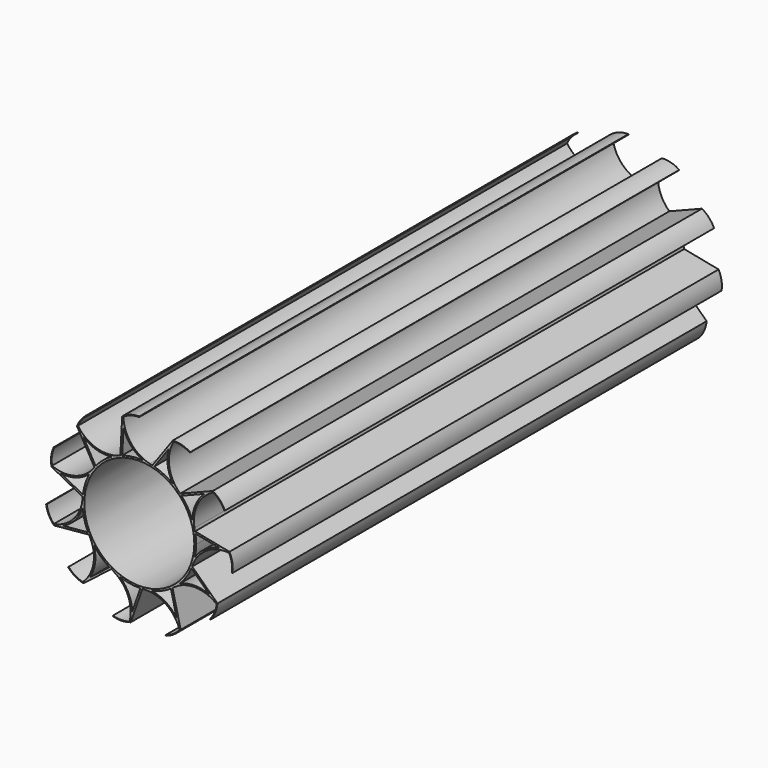
from build123d import *

# Parameters (mm, degrees)
F0_R          = 450
F1_DEPTH      = 5000
F4_DEPTH      = 7
F4_DEPTH_BACK = 7


# Not quite as in the source:
# - a feature names something its author has since deleted; it is built from what else it names


with BuildPart() as f1:
    # F0 (on Front) → F1 (new body)
    with BuildSketch(Plane.XZ):
        with BuildLine():
            ThreePointArc((29.6722661009, 464.0523209989), (57.272095407, 461.4595400332), (84.6683771855, 457.226711714))
            ThreePointArc((84.6683771855, 457.226711714), (-67.5951607035, 555.0944140008), (-130, 725))
            ThreePointArc((-130, 725), (-68.0073525437, 754.773895767), (0, 765))
            Line((0, 765), (0, 770))
            ThreePointArc((0, 770), (-73.5272058493, 758.4735293088), (-140, 725))
            Line((-140, 725), (-154.7293809103, 438.5017886886))
            ThreePointArc((-154.7293809103, 438.5017886886), (-147.110538763, 441.1161858115), (-139.4475537059, 443.5982188484))
            Line((-139.4475537059, 443.5982188484), (-129.0431979691, 645.9712395866))
            ThreePointArc((-129.0431979691, 645.9712395866), (-68.9398579749, 538.2132538291), (29.6722661009, 464.0523209989))
        make_face()
        with BuildLine():
            ThreePointArc((455.106133728, -95.4117762291), (462.5199196702, -47.9616920912), (465, 0))
            ThreePointArc((465, 0), (463.4796356702, 37.5716291765), (458.9284846496, 74.8975699022))
            ThreePointArc((458.9284846496, 74.8975699022), (457.5622716093, 82.8357869508), (456.0587595675, 90.7491477743))
            ThreePointArc((456.0587595675, 90.7491477743), (453.3481669029, 101.785731934), (451.0805611151, 112.9217755089))
            ThreePointArc((451.0805611151, 112.9217755089), (443.550050434, 139.6006903996), (434.4431435072, 165.7834583413))
            ThreePointArc((434.4431435072, 165.7834583413), (396.7252572047, 242.5573546522), (345.5825256109, 311.1233163753))
            ThreePointArc((345.5825256109, 311.1233163753), (340.1414699099, 317.0627389769), (334.5983492287, 322.9070217469))
            ThreePointArc((334.5983492287, 322.9070217469), (326.3512256914, 330.7261301277), (318.4229946099, 338.86840588))
            ThreePointArc((318.4229946099, 338.86840588), (297.66421554, 357.2408358334), (275.8475248515, 374.3436162583))
            ThreePointArc((275.8475248515, 374.3436162583), (202.6101176878, 418.5380988758), (122.5165564603, 448.5696081915))
            ThreePointArc((122.5165564603, 448.5696081915), (114.7281548389, 450.6245116361), (106.9053271687, 452.5441978668))
            ThreePointArc((106.9053271687, 452.5441978668), (95.7400762106, 454.6633188049), (84.6683771855, 457.226711714))
            ThreePointArc((84.6683771855, 457.226711714), (57.272095407, 461.4595400332), (29.6722661009, 464.0523209989))
            ThreePointArc((29.6722661009, 464.0523209989), (-55.8323026203, 461.6359539552), (-139.4475537059, 443.5982188484))
            ThreePointArc((-139.4475537059, 443.5982188484), (-147.110538763, 441.1161858115), (-154.7293809103, 438.5017886886))
            ThreePointArc((-154.7293809103, 438.5017886886), (-165.2678710001, 434.2481162591), (-175.9678517572, 430.4187671883))
            ThreePointArc((-175.9678517572, 430.4187671883), (-201.3035103525, 419.1681007899), (-225.9237274825, 406.4276926593))
            ThreePointArc((-225.9237274825, 406.4276926593), (-296.5483613387, 358.1676554176), (-357.1380508598, 297.7875293361))
            ThreePointArc((-357.1380508598, 297.7875293361), (-362.2426757411, 291.5565877697), (-367.238603816, 285.2381599073))
            ThreePointArc((-367.238603816, 285.2381599073), (-373.8044368952, 275.9622050517), (-380.7355310964, 266.9559052741))
            ThreePointArc((-380.7355310964, 266.9559052741), (-395.9666739177, 243.793751246), (-409.790533891, 219.7651435813))
            ThreePointArc((-409.790533891, 219.7651435813), (-443.1124106426, 140.9836569767), (-461.4397402826, 57.4314033257))
            ThreePointArc((-461.4397402826, 57.4314033257), (-462.3653226558, 49.4298331515), (-463.152164794, 41.413430752))
            ThreePointArc((-463.152164794, 41.413430752), (-463.6607352521, 30.060243596), (-464.6223694612, 18.7364296556))
            ThreePointArc((-464.6223694612, 18.7364296556), (-464.9132162808, -8.9833917542), (-463.5517412306, -36.6712857975))
            ThreePointArc((-463.5517412306, -36.6712857975), (-448.9914004502, -120.9616564115), (-419.237572543, -201.1587874497))
            ThreePointArc((-419.237572543, -201.1587874497), (-415.6902465446, -208.3905442378), (-412.0181859267, -215.5597700538))
            ThreePointArc((-412.0181859267, -215.5597700538), (-406.3080262366, -225.3856328058), (-400.9948883869, -235.4317299933))
            ThreePointArc((-400.9948883869, -235.4317299933), (-386.2530973946, -258.908371346), (-370.1385460296, -281.4648410425))
            ThreePointArc((-370.1385460296, -281.4648410425), (-312.3187930364, -344.5024985632), (-243.9304377122, -395.8824845298))
            ThreePointArc((-243.9304377122, -395.8824845298), (-237.0364542824, -400.0483962488), (-230.0713442091, -404.09426694))
            ThreePointArc((-230.0713442091, -404.09426694), (-219.9553897263, -409.2731632906), (-210.0543635442, -414.8519788504))
            ThreePointArc((-210.0543635442, -414.8519788504), (-184.9603492196, -426.6317723946), (-159.2089777382, -436.895297992))
            ThreePointArc((-159.2089777382, -436.895297992), (-76.4871755728, -458.6662315594), (8.8228875621, -464.9162899438))
            ThreePointArc((8.8228875621, -464.9162899438), (16.874737395, -464.6937090578), (24.9215236884, -464.3316892665))
            ThreePointArc((24.9215236884, -464.3316892665), (36.2315288916, -463.2193562166), (47.5769375506, -462.5596556265))
            ThreePointArc((47.5769375506, -462.5596556265), (75.0560029652, -458.902600144), (102.2683160682, -453.6145847838))
            ThreePointArc((102.2683160682, -453.6145847838), (183.6285797026, -427.2066768163), (258.775008375, -386.3424582421))
            ThreePointArc((258.775008375, -386.3424582421), (265.4283191806, -381.8020526097), (272.001983902, -377.1470810617))
            ThreePointArc((272.001983902, -377.1470810617), (280.9151930861, -370.0966764954), (290.1028971356, -363.4079100316))
            ThreePointArc((290.1028971356, -363.4079100316), (311.242604529, -345.4750947984), (331.2761421164, -326.3144459942))
            ThreePointArc((331.2761421164, -326.3144459942), (385.4435583801, -260.1120206821), (426.5678924457, -185.1076258139))
            ThreePointArc((426.5678924457, -185.1076258139), (429.7102850532, -177.6909421425), (432.7237361008, -170.2209394138))
            ThreePointArc((432.7237361008, -170.2209394138), (436.4102683277, -159.4709169651), (440.5232366492, -148.8767207192))
            ThreePointArc((440.5232366492, -148.8767207192), (448.61187829, -122.3616878648), (455.106133728, -95.4117762291))
        make_face()
        Circle(F0_R, mode=Mode.SUBTRACT)
        with BuildLine():
            ThreePointArc((456.0587595675, 90.7491477743), (457.5622716093, 82.8357869508), (458.9284846496, 74.8975699022))
            Line((458.9284846496, 74.8975699022), (657.7609456305, 35.7984317878))
            ThreePointArc((657.7609456305, 35.7984317878), (542.5461836828, -8.3575825515), (455.106133728, -95.4117762291))
            ThreePointArc((455.106133728, -95.4117762291), (448.61187829, -122.3616878648), (440.5232366492, -148.8767207192))
            ThreePointArc((440.5232366492, -148.8767207192), (559.0641476099, -12.0910323233), (736.1214743392, 25.4985296964))
            ThreePointArc((736.1214743392, 25.4985296964), (756.7698411808, -40.1003891557), (757.2134030389, -108.8708512791))
            Line((757.2134030389, -108.8708512791), (762.1625102483, -109.5824254704))
            ThreePointArc((762.1625102483, -109.5824254704), (761.2173748181, -35.163232747), (737.5446227219, 35.3967441152))
            Line((737.5446227219, 35.3967441152), (456.0587595675, 90.7491477743))
        make_face()
        with BuildLine():
            ThreePointArc((434.4431435072, 165.7834583413), (443.550050434, 139.6006903996), (451.0805611151, 112.9217755089))
            ThreePointArc((451.0805611151, 112.9217755089), (476.8515948552, 292.0812741164), (605.4792449418, 419.4280438225))
            ThreePointArc((605.4792449418, 419.4280438225), (658.3152096068, 375.4060715166), (695.8684764462, 317.7924849464))
            Line((695.8684764462, 317.7924849464), (700.416636423, 319.8695600115))
            ThreePointArc((700.416636423, 319.8695600115), (659.3874847149, 381.9639900089), (601.3250948118, 428.524363776))
            Line((601.3250948118, 428.524363776), (334.5983492287, 322.9070217469))
            ThreePointArc((334.5983492287, 322.9070217469), (340.1414699099, 317.0627389769), (345.5825256109, 311.1233163753))
            Line((345.5825256109, 311.1233163753), (533.9896258446, 385.7279725473))
            ThreePointArc((533.9896258446, 385.7279725473), (460.9373440098, 286.2917664064), (434.4431435072, 165.7834583413))
        make_face()
        with BuildLine():
            Line((639.5989441592, -368.9690917007), (432.7237361008, -170.2209394138))
            ThreePointArc((432.7237361008, -170.2209394138), (429.7102850532, -177.6909421425), (426.5678924457, -185.1076258139))
            Line((426.5678924457, -185.1076258139), (572.6978126954, -325.4968581247))
            ThreePointArc((572.6978126954, -325.4968581247), (451.9004434847, -300.353458101), (331.2761421164, -326.3144459942))
            ThreePointArc((331.2761421164, -326.3144459942), (311.242604529, -345.4750947984), (290.1028971356, -363.4079100316))
            ThreePointArc((290.1028971356, -363.4079100316), (463.777783657, -312.4245214315), (633.0503368197, -376.5265874443))
            ThreePointArc((633.0503368197, -376.5265874443), (614.95539526, -442.8752596068), (578.148424381, -500.9684614681))
            Line((578.148424381, -500.9684614681), (581.9271722528, -504.2427651379))
            ThreePointArc((581.9271722528, -504.2427651379), (621.3661269215, -441.1263775572), (639.5989441592, -368.9690917007))
        make_face()
        with BuildLine():
            Line((338.5851200161, -656.1898479127), (272.001983902, -377.1470810617))
            ThreePointArc((272.001983902, -377.1470810617), (265.4283191806, -381.8020526097), (258.775008375, -386.3424582421))
            Line((258.775008375, -386.3424582421), (305.8071707189, -583.4491954336))
            ThreePointArc((305.8071707189, -583.4491954336), (217.7795054561, -496.9892328997), (102.2683160682, -453.6145847838))
            ThreePointArc((102.2683160682, -453.6145847838), (75.0560029652, -458.902600144), (47.5769375506, -462.5596556265))
            ThreePointArc((47.5769375506, -462.5596556265), (221.2452502902, -513.5654324714), (328.9901902799, -659.0071734811))
            ThreePointArc((328.9901902799, -659.0071734811), (277.8969564114, -705.0403643399), (215.5254059837, -734.0121248151))
            Line((215.5254059837, -734.0121248151), (216.9340687679, -738.8095896832))
            ThreePointArc((216.9340687679, -738.8095896832), (284.2355240906, -707.0350143431), (338.5851200161, -656.1898479127))
        make_face()
        with BuildLine():
            Line((-69.927087404, -735.0749638283), (24.9215236884, -464.3316892665))
            ThreePointArc((24.9215236884, -464.3316892665), (16.874737395, -464.6937090578), (8.8228875621, -464.9162899438))
            Line((8.8228875621, -464.9162899438), (-58.1750872306, -656.1605356472))
            ThreePointArc((-58.1750872306, -656.1605356472), (-85.4848867983, -535.8344378108), (-159.2089777382, -436.895297992))
            ThreePointArc((-159.2089777382, -436.895297992), (-184.9603492196, -426.6317723946), (-210.0543635442, -414.8519788504))
            ThreePointArc((-210.0543635442, -414.8519788504), (-91.5310867995, -551.6529473815), (-79.5220171402, -732.2576382599))
            ThreePointArc((-79.5220171402, -732.2576382599), (-147.3918025718, -743.3601349722), (-215.5254059837, -734.0121248151))
            Line((-215.5254059837, -734.0121248151), (-216.9340687679, -738.8095896832))
            ThreePointArc((-216.9340687679, -738.8095896832), (-143.1378493268, -748.4650297457), (-69.927087404, -735.0749638283))
        make_face()
        with BuildLine():
            Line((-456.2379386545, -580.5789725199), (-230.0713442091, -404.09426694))
            ThreePointArc((-230.0713442091, -404.09426694), (-237.0364542824, -400.0483962488), (-243.9304377122, -395.8824845298))
            Line((-243.9304377122, -395.8824845298), (-403.68716603, -520.5455420017))
            ThreePointArc((-403.68716603, -520.5455420017), (-361.6084315016, -404.5559947422), (-370.1385460296, -281.4648410425))
            ThreePointArc((-370.1385460296, -281.4648410425), (-386.2530973946, -258.908371346), (-400.9948883869, -235.4317299933))
            ThreePointArc((-400.9948883869, -235.4317299933), (-375.2469505581, -414.5945492916), (-462.786545994, -573.0214767764))
            ThreePointArc((-462.786545994, -573.0214767764), (-525.8847056592, -545.6683150825), (-578.148424381, -500.9684614681))
            Line((-578.148424381, -500.9684614681), (-581.9271722528, -504.2427651379))
            ThreePointArc((-581.9271722528, -504.2427651379), (-525.0659669467, -552.2626866053), (-456.2379386545, -580.5789725199))
        make_face()
        with BuildLine():
            Line((-697.6964680054, -241.7532596115), (-412.0181859267, -215.5597700538))
            ThreePointArc((-412.0181859267, -215.5597700538), (-415.6902465446, -208.3905442378), (-419.237572543, -201.1587874497))
            Line((-419.237572543, -201.1587874497), (-621.031421932, -219.6610167697))
            ThreePointArc((-621.031421932, -219.6610167697), (-522.9238542063, -144.833881799), (-463.5517412306, -36.6712857975))
            ThreePointArc((-463.5517412306, -36.6712857975), (-464.9132162808, -8.9833917542), (-464.6223694612, 18.7364296556))
            ThreePointArc((-464.6223694612, 18.7364296556), (-539.8245588828, -145.9053111866), (-699.1196163881, -231.8550451927))
            ThreePointArc((-699.1196163881, -231.8550451927), (-737.4129304235, -174.7306606623), (-757.2134030389, -108.8708512791))
            Line((-757.2134030389, -108.8708512791), (-762.1625102483, -109.5824254704))
            ThreePointArc((-762.1625102483, -109.5824254704), (-740.2893499999, -180.7208425693), (-697.6964680054, -241.7532596115))
        make_face()
        with BuildLine():
            ThreePointArc((-409.790533891, 219.7651435813), (-395.9666739177, 243.793751246), (-380.7355310964, 266.9559052741))
            ThreePointArc((-380.7355310964, 266.9559052741), (-533.0116839802, 169.1078323024), (-713.4871483223, 182.9237250303))
            ThreePointArc((-713.4871483223, 182.9237250303), (-714.8177600892, 251.6827439304), (-695.8684764462, 317.7924849464))
            Line((-695.8684764462, 317.7924849464), (-700.416636423, 319.8695600115))
            ThreePointArc((-700.416636423, 319.8695600115), (-720.4760950626, 248.1985920699), (-717.6412984523, 173.8274050767))
            Line((-717.6412984523, 173.8274050767), (-463.152164794, 41.413430752))
            ThreePointArc((-463.152164794, 41.413430752), (-462.3653226558, 49.4298331515), (-461.4397402826, 57.4314033257))
            Line((-461.4397402826, 57.4314033257), (-641.2025893689, 150.9643292361))
            ThreePointArc((-641.2025893689, 150.9643292361), (-518.2146480038, 160.8719652681), (-409.790533891, 219.7651435813))
        make_face()
        with BuildLine():
            ThreePointArc((-225.9237274825, 406.4276926593), (-201.3035103525, 419.1681007899), (-175.9678517572, 430.4187671883))
            ThreePointArc((-175.9678517572, 430.4187671883), (-356.9713654945, 430.4304338943), (-501.3275519234, 539.6255050334))
            ThreePointArc((-501.3275519234, 539.6255050334), (-465.2730015875, 598.1886556305), (-413.5902253535, 643.5589526159))
            Line((-413.5902253535, 643.5589526159), (-416.2934294408, 647.76522028))
            ThreePointArc((-416.2934294408, 647.76522028), (-471.9167705839, 598.3167274144), (-509.7400872517, 534.2190968588))
            Line((-509.7400872517, 534.2190968588), (-367.238603816, 285.2381599073))
            ThreePointArc((-367.238603816, 285.2381599073), (-362.2426757411, 291.5565877697), (-357.1380508598, 297.7875293361))
            Line((-357.1380508598, 297.7875293361), (-457.7964652023, 473.6595673725))
            ThreePointArc((-457.7964652023, 473.6595673725), (-348.9759525899, 415.5021000295), (-225.9237274825, 406.4276926593))
        make_face()
        with BuildLine():
            ThreePointArc((275.8475248515, 374.3436162583), (297.66421554, 357.2408358334), (318.4229946099, 338.86840588))
            ThreePointArc((318.4229946099, 338.86840588), (243.2420300064, 503.5198397718), (282.6016333873, 680.1921175718))
            ThreePointArc((282.6016333873, 680.1921175718), (350.8501504157, 671.7237569749), (413.5902253535, 643.5589526159))
            Line((413.5902253535, 643.5589526159), (416.2934294408, 647.76522028))
            ThreePointArc((416.2934294408, 647.76522028), (348.2067272241, 677.8203447656), (274.1890980589, 685.5985257464))
            Line((274.1890980589, 685.5985257464), (106.9053271687, 452.5441978668))
            ThreePointArc((106.9053271687, 452.5441978668), (114.7281548389, 450.6245116361), (122.5165564603, 448.5696081915))
            Line((122.5165564603, 448.5696081915), (240.6803728435, 613.1916074467))
            ThreePointArc((240.6803728435, 613.1916074467), (232.9841544413, 490.0455023711), (275.8475248515, 374.3436162583))
        make_face()
    extrude(amount=F1_DEPTH)

    # F3 (on offset) → F4 (join, two sides)
    with BuildSketch(Plane.XZ.offset(2500)) as f4_sk:
        with BuildLine():
            ThreePointArc((7, 449.9455522616), (0, 450), (-7, 449.9455522616))
            ThreePointArc((-7, 449.9455522616), (-5.9827295721, 442.2047696555), (-3, 434.9896550494))
            ThreePointArc((-3, 434.9896550494), (0, 434.6927972661), (3, 434.9896550494))
            ThreePointArc((3, 434.9896550494), (5.9827295721, 442.2047696555), (7, 449.9455522616))
        make_face()
        with BuildLine():
            ThreePointArc((-137.2723653364, 412.7726949726), (-134.3274616876, 413.4174174265), (-131.5660262387, 414.6267969388))
            ThreePointArc((-131.5660262387, 414.6267969388), (-130.9588748724, 422.4104928282), (-132.3834265782, 430.086768417))
            ThreePointArc((-132.3834265782, 430.086768417), (-139.0576474687, 427.9754323328), (-145.6982178063, 425.7605304958))
            ThreePointArc((-145.6982178063, 425.7605304958), (-142.338702762, 418.7129626071), (-137.2723653364, 412.7726949726))
        make_face()
        with BuildLine():
            ThreePointArc((-258.107555121, 350.1506675554), (-255.5060155108, 351.6738603207), (-253.2534531547, 353.6773790691))
            ThreePointArc((-253.2534531547, 353.6773790691), (-255.0813122003, 361.2677338559), (-258.8082409933, 368.1280950891))
            ThreePointArc((-258.8082409933, 368.1280950891), (-264.5033635316, 364.0576474687), (-270.1344789146, 359.899101557))
            ThreePointArc((-270.1344789146, 359.899101557), (-264.7615719935, 354.234613434), (-258.107555121, 350.1506675554))
        make_face()
        with BuildLine():
            ThreePointArc((-353.6773790691, 253.2534531547), (-351.6738603207, 255.5060155108), (-350.1506675554, 258.107555121))
            ThreePointArc((-350.1506675554, 258.107555121), (-354.234613434, 264.7615719935), (-359.899101557, 270.1344789146))
            ThreePointArc((-359.899101557, 270.1344789146), (-364.0576474687, 264.5033635316), (-368.1280950891, 258.8082409933))
            ThreePointArc((-368.1280950891, 258.8082409933), (-361.2677338559, 255.0813122003), (-353.6773790691, 253.2534531547))
        make_face()
        with BuildLine():
            ThreePointArc((-414.6267969388, 131.5660262387), (-413.4174174265, 134.3274616876), (-412.7726949726, 137.2723653364))
            ThreePointArc((-412.7726949726, 137.2723653364), (-418.7129626071, 142.338702762), (-425.7605304958, 145.6982178063))
            ThreePointArc((-425.7605304958, 145.6982178063), (-427.9754323328, 139.0576474687), (-430.086768417, 132.3834265782))
            ThreePointArc((-430.086768417, 132.3834265782), (-422.4104928282, 130.9588748724), (-414.6267969388, 131.5660262387))
        make_face()
        with BuildLine():
            ThreePointArc((-434.9896550494, -3), (-434.6927972661, 0), (-434.9896550494, 3))
            ThreePointArc((-434.9896550494, 3), (-442.2047696555, 5.9827295721), (-449.9455522616, 7))
            ThreePointArc((-449.9455522616, 7), (-450, 0), (-449.9455522616, -7))
            ThreePointArc((-449.9455522616, -7), (-442.2047696555, -5.9827295721), (-434.9896550494, -3))
        make_face()
        with BuildLine():
            ThreePointArc((-412.7726949726, -137.2723653364), (-413.4174174265, -134.3274616876), (-414.6267969388, -131.5660262387))
            ThreePointArc((-414.6267969388, -131.5660262387), (-422.4104928282, -130.9588748724), (-430.086768417, -132.3834265782))
            ThreePointArc((-430.086768417, -132.3834265782), (-427.9754323328, -139.0576474687), (-425.7605304958, -145.6982178063))
            ThreePointArc((-425.7605304958, -145.6982178063), (-418.7129626071, -142.338702762), (-412.7726949726, -137.2723653364))
        make_face()
        with BuildLine():
            ThreePointArc((-350.1506675554, -258.107555121), (-351.6738603207, -255.5060155108), (-353.6773790691, -253.2534531547))
            ThreePointArc((-353.6773790691, -253.2534531547), (-361.2677338559, -255.0813122003), (-368.1280950891, -258.8082409933))
            ThreePointArc((-368.1280950891, -258.8082409933), (-364.0576474687, -264.5033635316), (-359.899101557, -270.1344789146))
            ThreePointArc((-359.899101557, -270.1344789146), (-354.234613434, -264.7615719935), (-350.1506675554, -258.107555121))
        make_face()
        with BuildLine():
            ThreePointArc((-253.2534531547, -353.6773790691), (-255.5060155108, -351.6738603207), (-258.107555121, -350.1506675554))
            ThreePointArc((-258.107555121, -350.1506675554), (-264.7615719935, -354.234613434), (-270.1344789146, -359.899101557))
            ThreePointArc((-270.1344789146, -359.899101557), (-264.5033635316, -364.0576474687), (-258.8082409933, -368.1280950891))
            ThreePointArc((-258.8082409933, -368.1280950891), (-255.0813122003, -361.2677338559), (-253.2534531547, -353.6773790691))
        make_face()
        with BuildLine():
            ThreePointArc((-131.5660262387, -414.6267969388), (-134.3274616876, -413.4174174265), (-137.2723653364, -412.7726949726))
            ThreePointArc((-137.2723653364, -412.7726949726), (-142.338702762, -418.7129626071), (-145.6982178063, -425.7605304958))
            ThreePointArc((-145.6982178063, -425.7605304958), (-139.0576474687, -427.9754323328), (-132.3834265782, -430.086768417))
            ThreePointArc((-132.3834265782, -430.086768417), (-130.9588748724, -422.4104928282), (-131.5660262387, -414.6267969388))
        make_face()
        with BuildLine():
            ThreePointArc((3, -434.9896550494), (0, -434.6927972661), (-3, -434.9896550494))
            ThreePointArc((-3, -434.9896550494), (-5.9827295721, -442.2047696555), (-7, -449.9455522616))
            ThreePointArc((-7, -449.9455522616), (0, -450), (7, -449.9455522616))
            ThreePointArc((7, -449.9455522616), (5.9827295721, -442.2047696555), (3, -434.9896550494))
        make_face()
        with BuildLine():
            ThreePointArc((137.2723653364, -412.7726949726), (134.3274616876, -413.4174174265), (131.5660262387, -414.6267969388))
            ThreePointArc((131.5660262387, -414.6267969388), (130.9588748724, -422.4104928282), (132.3834265782, -430.086768417))
            ThreePointArc((132.3834265782, -430.086768417), (139.0576474687, -427.9754323328), (145.6982178063, -425.7605304958))
            ThreePointArc((145.6982178063, -425.7605304958), (142.338702762, -418.7129626071), (137.2723653364, -412.7726949726))
        make_face()
        with BuildLine():
            ThreePointArc((258.107555121, -350.1506675554), (255.5060155108, -351.6738603207), (253.2534531547, -353.6773790691))
            ThreePointArc((253.2534531547, -353.6773790691), (255.0813122003, -361.2677338559), (258.8082409933, -368.1280950891))
            ThreePointArc((258.8082409933, -368.1280950891), (264.5033635316, -364.0576474687), (270.1344789146, -359.899101557))
            ThreePointArc((270.1344789146, -359.899101557), (264.7615719935, -354.234613434), (258.107555121, -350.1506675554))
        make_face()
        with BuildLine():
            ThreePointArc((353.6773790691, -253.2534531547), (351.6738603207, -255.5060155108), (350.1506675554, -258.107555121))
            ThreePointArc((350.1506675554, -258.107555121), (354.234613434, -264.7615719935), (359.899101557, -270.1344789146))
            ThreePointArc((359.899101557, -270.1344789146), (364.0576474687, -264.5033635316), (368.1280950891, -258.8082409933))
            ThreePointArc((368.1280950891, -258.8082409933), (361.2677338559, -255.0813122003), (353.6773790691, -253.2534531547))
        make_face()
        with BuildLine():
            ThreePointArc((414.6267969388, -131.5660262387), (413.4174174265, -134.3274616876), (412.7726949726, -137.2723653364))
            ThreePointArc((412.7726949726, -137.2723653364), (418.7129626071, -142.338702762), (425.7605304958, -145.6982178063))
            ThreePointArc((425.7605304958, -145.6982178063), (427.9754323328, -139.0576474687), (430.086768417, -132.3834265782))
            ThreePointArc((430.086768417, -132.3834265782), (422.4104928282, -130.9588748724), (414.6267969388, -131.5660262387))
        make_face()
        with BuildLine():
            ThreePointArc((434.9896550494, 3), (434.6927972661, 0), (434.9896550494, -3))
            ThreePointArc((434.9896550494, -3), (442.2047696555, -5.9827295721), (449.9455522616, -7))
            ThreePointArc((449.9455522616, -7), (450, 0), (449.9455522616, 7))
            ThreePointArc((449.9455522616, 7), (442.2047696555, 5.9827295721), (434.9896550494, 3))
        make_face()
        with BuildLine():
            ThreePointArc((412.7726949726, 137.2723653364), (413.4174174265, 134.3274616876), (414.6267969388, 131.5660262387))
            ThreePointArc((414.6267969388, 131.5660262387), (422.4104928282, 130.9588748724), (430.086768417, 132.3834265782))
            ThreePointArc((430.086768417, 132.3834265782), (427.9754323328, 139.0576474687), (425.7605304958, 145.6982178063))
            ThreePointArc((425.7605304958, 145.6982178063), (418.7129626071, 142.338702762), (412.7726949726, 137.2723653364))
        make_face()
        with BuildLine():
            ThreePointArc((350.1506675554, 258.107555121), (351.6738603207, 255.5060155108), (353.6773790691, 253.2534531547))
            ThreePointArc((353.6773790691, 253.2534531547), (361.2677338559, 255.0813122003), (368.1280950891, 258.8082409933))
            ThreePointArc((368.1280950891, 258.8082409933), (364.0576474687, 264.5033635316), (359.899101557, 270.1344789146))
            ThreePointArc((359.899101557, 270.1344789146), (354.234613434, 264.7615719935), (350.1506675554, 258.107555121))
        make_face()
        with BuildLine():
            ThreePointArc((253.2534531547, 353.6773790691), (255.5060155108, 351.6738603207), (258.107555121, 350.1506675554))
            ThreePointArc((258.107555121, 350.1506675554), (264.7615719935, 354.234613434), (270.1344789146, 359.899101557))
            ThreePointArc((270.1344789146, 359.899101557), (264.5033635316, 364.0576474687), (258.8082409933, 368.1280950891))
            ThreePointArc((258.8082409933, 368.1280950891), (255.0813122003, 361.2677338559), (253.2534531547, 353.6773790691))
        make_face()
        with BuildLine():
            ThreePointArc((131.5660262387, 414.6267969388), (134.3274616876, 413.4174174265), (137.2723653364, 412.7726949726))
            ThreePointArc((137.2723653364, 412.7726949726), (142.338702762, 418.7129626071), (145.6982178063, 425.7605304958))
            ThreePointArc((145.6982178063, 425.7605304958), (139.0576474687, 427.9754323328), (132.3834265782, 430.086768417))
            ThreePointArc((132.3834265782, 430.086768417), (130.9588748724, 422.4104928282), (131.5660262387, 414.6267969388))
        make_face()
    extrude(amount=F4_DEPTH)
    extrude(f4_sk.sketch, amount=-F4_DEPTH_BACK)


solid = f1.part
